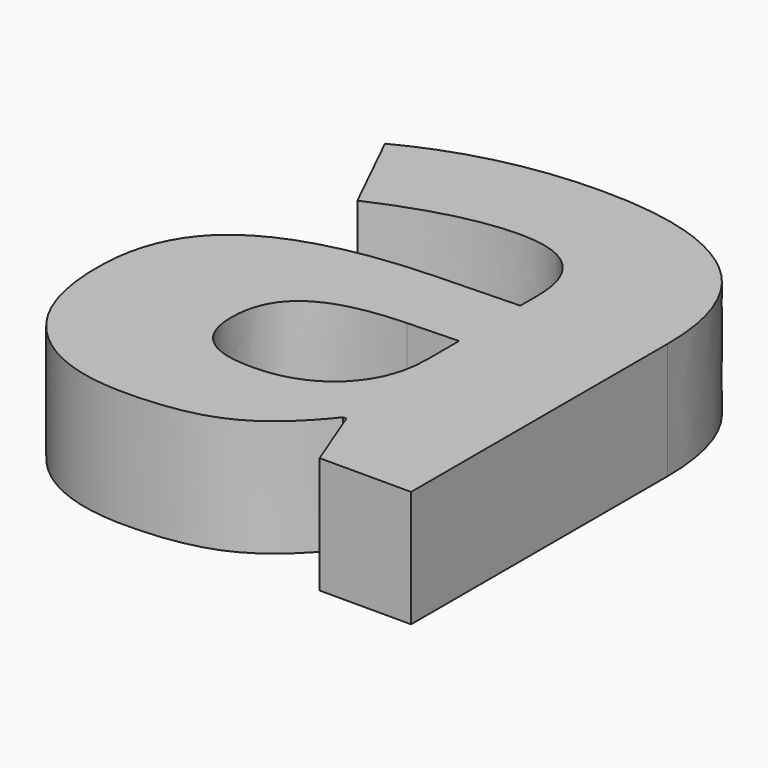
from build123d import *

# Parameters (mm, degrees)
F0_TEXT_SIZE = 75.5299400124
F1_DEPTH     = 10


# Not quite as in the source:
# - Text() gives the source's letters only with a copy of the font that has no kerning and outlines rounded to 1/6400 em; it was checked with that copy


with BuildPart() as f1:
    # F0 (on Top) → F1 (new body)
    with BuildSketch(Plane.XY):
        with Locations((0, 0)):
            Text('a', F0_TEXT_SIZE, font='Open Sans', font_style=FontStyle.BOLD, text_align=(TextAlign.LEFT, TextAlign.BOTTOM))
    extrude(amount=F1_DEPTH)


solid = f1.part
